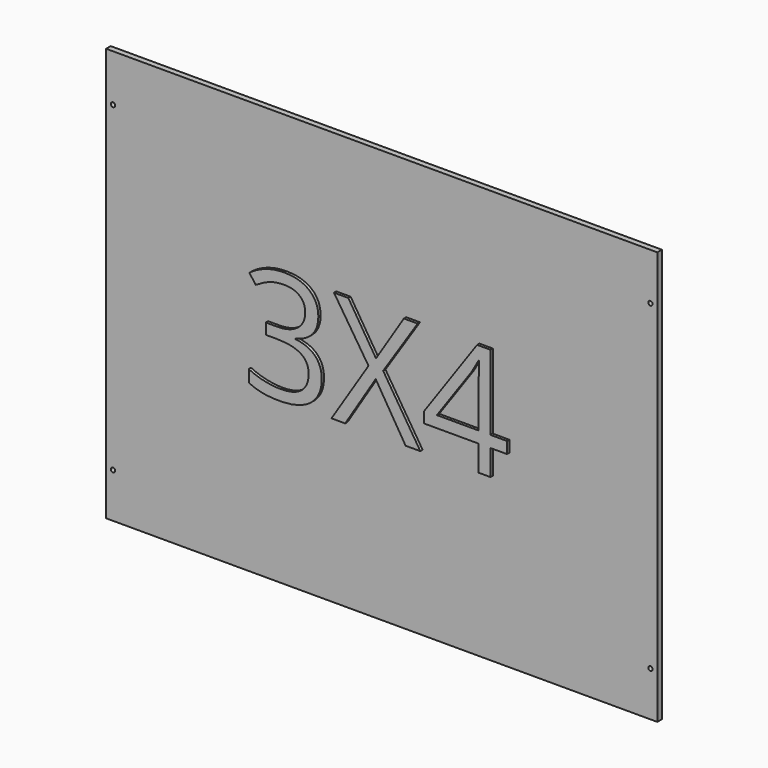
from build123d import *

# Parameters (mm, degrees)
F0_W         = 1219.2
F0_H         = 914.4
F1_DEPTH     = 12.7
F2_R         = 4.7625
F3_DEPTH     = 12.701
F4_TEXT_SIZE = 345.2907336932
F5_DEPTH     = 6.35
F6_TEXT_SIZE = 345.2907336932
F7_DEPTH     = 6.35


# Not quite as in the source:
# - Text() gives the source's letters only with a copy of the font that has no kerning and outlines rounded to 1/6400 em; it was checked with that copy


with BuildPart() as f1:
    # F0 (on Front) → F1 (new body)
    with BuildSketch(Plane.XZ):
        with Locations((609.6, 457.2)):
            Rectangle(F0_W, F0_H)
    extrude(amount=F1_DEPTH)

    # F2 (on face) → F3 (cut, through all)
    with BuildSketch(Plane.XZ.offset(12.7)):
        with Locations((1203.96, 810.26)):
            Circle(F2_R)
        with Locations((1203.96, 99.06)):
            Circle(F2_R)
        with Locations((15.24, 99.06)):
            Circle(F2_R)
        with Locations((15.24, 810.26)):
            Circle(F2_R)
    extrude(amount=-F3_DEPTH, mode=Mode.SUBTRACT)

    # F4 (on face) → F5 (join)
    with BuildSketch(Plane.XZ.offset(12.7)):
        with Locations((304.8, 360.9906717409)):
            Text('3X4', F4_TEXT_SIZE, font='Open Sans', text_align=(TextAlign.LEFT, TextAlign.BOTTOM))
    extrude(amount=F5_DEPTH)

    # F6 (on face) → F7 (join)
    with BuildSketch(Plane(origin=(0, 0, 0), x_dir=(-1, 0, 0), z_dir=(0, 1, 0))):
        with Locations((-914.4, 360.9906717409)):
            Text('3X4', F6_TEXT_SIZE, font='Open Sans', text_align=(TextAlign.LEFT, TextAlign.BOTTOM))
    extrude(amount=F7_DEPTH)


solid = f1.part
